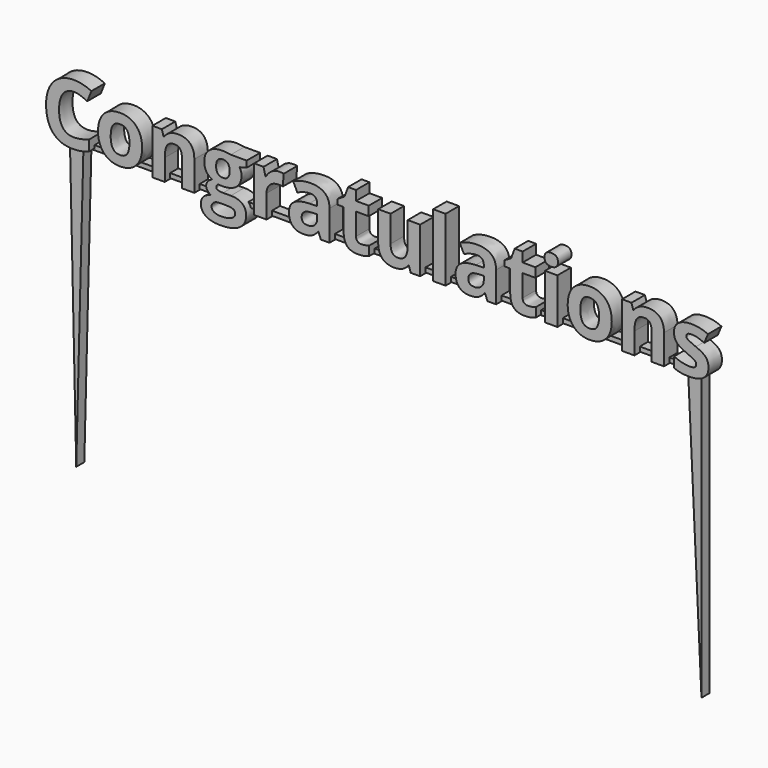
from build123d import *

# Parameters (mm, degrees)
F0_TEXT_SIZE = 6.2896829235
F1_DEPTH     = 1.27
F2_W         = 47.126153484
F2_H         = 0.343359774
F3_DEPTH     = 0.762
F5_DEPTH     = 0.762
F6_DEPTH     = 0.762


# Not quite as in the source:
# - Text() gives the source's letters only with a copy of the font that has no kerning and outlines rounded to 1/6400 em; it was checked with that copy


with BuildPart() as f1:
    # F0 (on Front) → F1 (new body)
    with BuildSketch(Plane.XZ):
        with Locations((-25.4, -2.1483940224)):
            Text('Congratulations', F0_TEXT_SIZE, font='Open Sans', font_style=FontStyle.BOLD, text_align=(TextAlign.LEFT, TextAlign.BOTTOM))
    extrude(amount=F1_DEPTH)


with BuildPart() as f3:
    # F2 (on Front) → F3 (new body)
    with BuildSketch(Plane.XZ):
        with Locations((0.1190090552, -1.9317235565)):
            Rectangle(F2_W, F2_H)
    extrude(amount=F3_DEPTH)


with BuildPart() as f5:
    # F4 (on Front) → F5 (new body)
    with BuildSketch(Plane.XZ):
        Polygon((-22.614043206, -2.0369556732), (-23.6395839602, -2.0369556732), (-23.1619738042, -23.5994104296), align=None)
    extrude(amount=F5_DEPTH)


with BuildPart() as f6:
    # F4 (on Front) → F6 (new body)
    with BuildSketch(Plane.XZ):
        Polygon((-22.614043206, -2.0369556732), (-23.6395839602, -2.0369556732), (-23.1619738042, -23.5994104296), align=None)
    extrude(amount=F6_DEPTH)


with BuildPart() as f6b:
    # F4 (on Front) → F6, piece 2 (new body)
    with BuildSketch(Plane.XZ):
        Polygon((24.0572784096, -2.0369556732), (23.0409633368, -2.0369556732), (24.0572784096, -23.5994104296), align=None)
    extrude(amount=F6_DEPTH)


solid = Compound([f1.part, f3.part, f5.part, f6.part, f6b.part])
